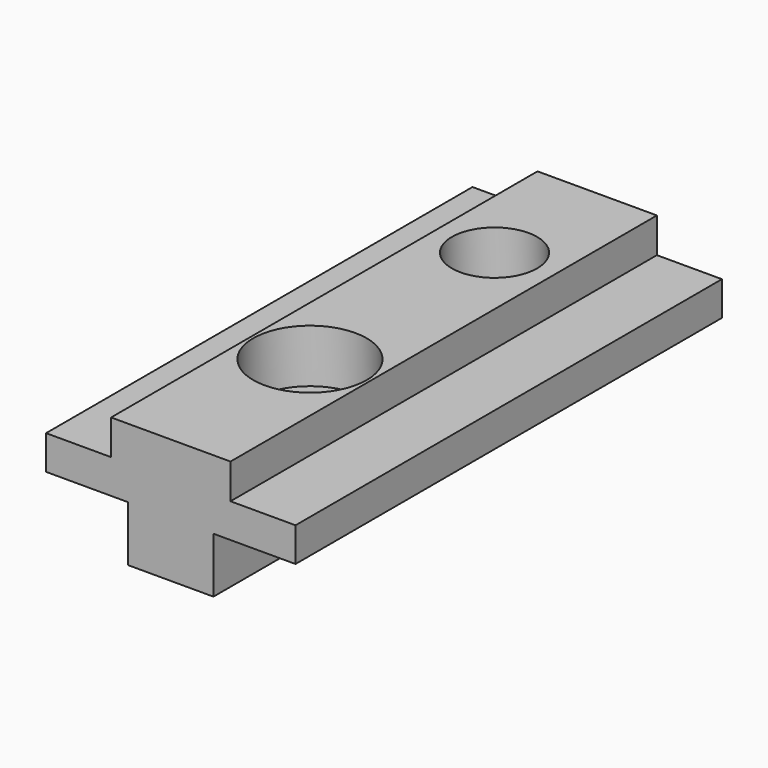
from build123d import *

# Parameters (mm, degrees)
F1_DEPTH = 31.75
F2_R     = 3.3782
F2_R_2   = 2.54
F3_DEPTH = 3.175


# Not quite as in the source:
# - a feature names something its author has since deleted; it is built from what else it names


with BuildPart() as f1:
    # F0 (on Front) → F1 (new body)
    with BuildSketch(Plane.XZ):
        Polygon((3.556, 2.0828), (-3.556, 2.0828), (-3.556, 0), (-7.4295, 0), (-7.4295, -2.032), (-2.54, -2.032), (-2.54, -5.334), (2.54, -5.334), (2.54, -2.032), (7.4295, -2.032), (7.4295, 0), (3.556, 0), align=None)
    extrude(amount=F1_DEPTH)

    # F2 (on face) → F3 (cut)
    with BuildSketch(Plane.XY.offset(2.0828)):
        with Locations((0, -21.3868)):
            Circle(F2_R)
        with Locations((0, -7.6454)):
            Circle(F2_R_2)
    extrude(amount=-F3_DEPTH, mode=Mode.SUBTRACT)


solid = f1.part
